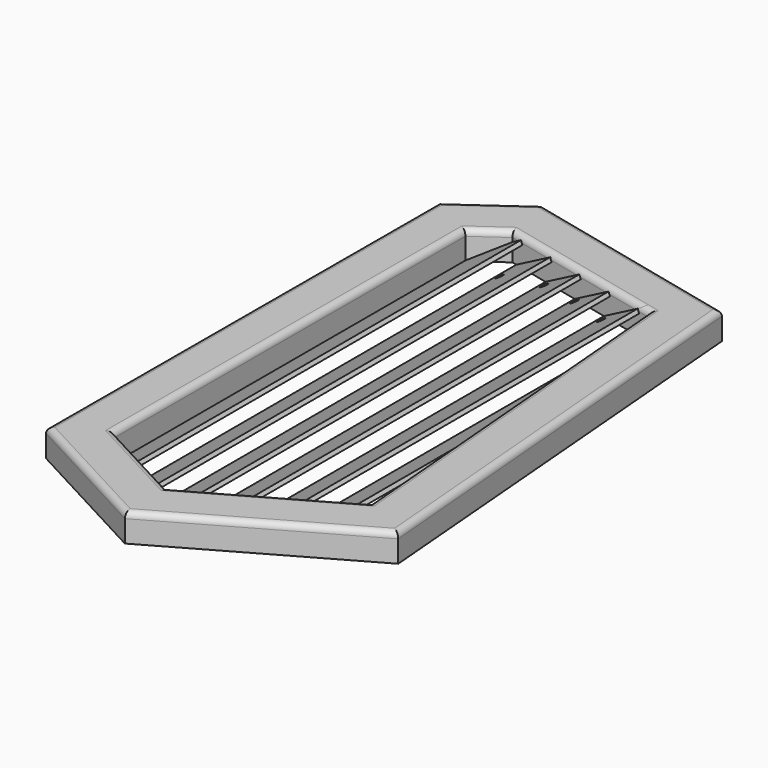
from build123d import *

# Parameters (mm, degrees)
F1_W           = 1
F1_H           = 127.4104844779
F2_DEPTH       = 12
F1_H_2         = 132.846667897
F1_H_3         = 133.8659538887
F1_H_4         = 125.3719197121
F1_H_5         = 118.236936396
F1_H_6         = 128.7695337087
F3_ANGLE       = -60
F4_ANGLE       = -60
F5_ANGLE       = -60
F6_ANGLE       = -60
F7_ANGLE       = -60
F8_ANGLE       = -60
F10_D          = 2
F12_D          = 2
F14_D          = 2
F16_D          = 2
F18_D          = 2
F19_DEPTH      = 7
F20_T1_DEPTH   = 64.3707659931
F20_T3_DEPTH   = 27.8907851503
F20_T5_DEPTH   = 130.1079313017
F20_T7_DEPTH   = 46.7691989997
F20_T9_DEPTH   = 61.7403046628
F20_T11_DEPTH  = 121.2232351314
F20_T16_DEPTH  = 47.9519770563
F20_T22_DEPTH  = 47.9519770563
F20_T28_DEPTH  = 47.9519770563
F20_T34_DEPTH  = 47.9519770563
F20_T40_DEPTH  = 47.9519770563
F20_T46_DEPTH  = 33.4399000359
F20_T52_DEPTH  = 33.4399000359
F20_T58_DEPTH  = 33.4399000359
F20_T64_DEPTH  = 117.2163729424
F20_T70_DEPTH  = 16.7204599427
F20_T76_DEPTH  = 50.7233823642
F20_T82_DEPTH  = 50.7233823642
F20_T88_DEPTH  = 50.7233823642
F20_T94_DEPTH  = 50.7233823642
F20_T100_DEPTH = 50.7233823642
F20_T106_DEPTH = 50.7233823642
F20_T112_DEPTH = 105.3966809672
F20_T118_DEPTH = 105.3966809672
F20_T125_DEPTH = 47.9519770563
F20_T129_DEPTH = 105.3966809672
F20_T136_DEPTH = 33.4399000359
F20_T140_DEPTH = 47.9519770563
F20_T147_DEPTH = 117.2163729424
F20_T151_DEPTH = 33.4399000359
F20_T158_DEPTH = 117.2163729424
F20_T162_DEPTH = 16.7204599427
F20_T169_DEPTH = 50.7233823642
F20_T173_DEPTH = 16.7204599427
F20_T180_DEPTH = 50.7233823642
F20_T184_DEPTH = 105.3966809672


# Not quite as in the source:
# - a fillet or chamfer that OpenCascade refuses, or shapes differently, is made with other operations: its cross-section is extruded or revolved along the edge and cut away or added


with BuildPart() as f2:
    # F1 (on Top) → F2 (new body)
    with BuildSketch(Plane.XY):
        with Locations((0.5, -55.8595443144)):
            Rectangle(F1_W, F1_H)
    extrude(amount=F2_DEPTH)


with BuildPart() as f2b:
    # F1 (on Top) → F2, piece 2 (new body)
    with BuildSketch(Plane.XY):
        with Locations((9.5, -58.9173960034)):
            Rectangle(F1_W, F1_H_2)
    extrude(amount=F2_DEPTH)


with BuildPart() as f2c:
    # F1 (on Top) → F2, piece 3 (new body)
    with BuildSketch(Plane.XY):
        with Locations((18.5, -60.1065598894)):
            Rectangle(F1_W, F1_H_3)
    extrude(amount=F2_DEPTH)


with BuildPart() as f2d:
    # F1 (on Top) → F2, piece 4 (new body)
    with BuildSketch(Plane.XY):
        with Locations((36.5, -59.257156332)):
            Rectangle(F1_W, F1_H_4)
    extrude(amount=F2_DEPTH)


with BuildPart() as f2e:
    # F1 (on Top) → F2, piece 5 (new body)
    with BuildSketch(Plane.XY):
        with Locations((45.5, -56.7089506658)):
            Rectangle(F1_W, F1_H_5)
    extrude(amount=F2_DEPTH)


with BuildPart() as f2f:
    # F1 (on Top) → F2, piece 6 (new body)
    with BuildSketch(Plane.XY):
        with Locations((27.5, -59.2571562156)):
            Rectangle(F1_W, F1_H_6)
    extrude(amount=F2_DEPTH)


with BuildPart() as f2_1:
    # F3: moved
    add(f2.part.rotate(Axis((0, -55.8595443144, 0), (0, -1, 0)), F3_ANGLE))



with BuildPart() as f2b_1:
    # F4: moved
    add(f2b.part.rotate(Axis((9, -58.9173960034, 0), (0, -1, 0)), F4_ANGLE))

    # F10 (through all)
    with Locations(Plane(origin=(2.25, 0, -3.897114317), x_dir=(0.8660254038, 0, 0.5), z_dir=(-0.5, 0, 0.8660254038))):
        with Locations((9.7942286341, -112.9602642174), (9.7942286341, -2.9387139806)):
            Hole(F10_D / 2)


with BuildPart() as f2c_1:
    # F5: moved
    add(f2c.part.rotate(Axis((18, -60.1065598894, 0), (0, -1, 0)), F5_ANGLE))

    # F12 (through all)
    with Locations(Plane(origin=(4.5, 0, -7.7942286341), x_dir=(0.8660254038, 0, 0.5), z_dir=(-0.5, 0, 0.8660254038))):
        with Locations((18.324283883, -117.2249242663), (18.324283883, -0.9955040878)):
            Hole(F12_D / 2)


with BuildPart() as f2f_1:
    # F6: moved
    add(f2f.part.rotate(Axis((27, -59.2571562156, 0), (0, -1, 0)), F6_ANGLE))

    # F14 (through all)
    with Locations(Plane(origin=(6.75, 0, -11.6913429511), x_dir=(0.8660254038, 0, 0.5), z_dir=(-0.5, 0, 0.8660254038))):
        with Locations((25.7820524275, -2.3019914515), (26.0747242719, -116.0897985101)):
            Hole(F14_D / 2)


with BuildPart() as f2d_1:
    # F7: moved
    add(f2d.part.rotate(Axis((36, -59.257156332, 0), (0, -1, 0)), F7_ANGLE))

    # F16 (through all)
    with Locations(Plane(origin=(9, 0, -15.5884572681), x_dir=(0.8660254038, 0, 0.5), z_dir=(-0.5, 0, 0.8660254038))):
        with Locations((33.6682610214, -110.1817563176), (33.4965772927, -5.2406745963)):
            Hole(F16_D / 2)


with BuildPart() as f2e_1:
    # F8: moved
    add(f2e.part.rotate(Axis((45, -56.7089506658, 0), (0, -1, 0)), F8_ANGLE))

    # F18 (through all)
    with Locations(Plane(origin=(11.25, 0, -19.4855715851), x_dir=(0.8660254038, 0, 0.5), z_dir=(-0.5, 0, 0.8660254038))):
        with Locations((41.2861332297, -6.0908603482), (41.4609648287, -105.8669760823)):
            Hole(F18_D / 2)


with BuildPart() as f2_2:
    add(f2_1.part)

    add(f2b_1.part)  # F19 merges F2b

    add(f2c_1.part)  # F19 merges F2c

    add(f2d_1.part)  # F19 merges F2d

    add(f2e_1.part)  # F19 merges F2e

    add(f2f_1.part)  # F19 merges F2f
    # F0 (on Top) → F19 (join)
    with BuildSketch(Plane.XY):
        Polygon((5.3426049832, 17.2253030222), (-11.2654683454, 5.3950021233), (-11.5938979585, -117.2124892957), (23.0112235707, -135.7746969778), (70.1950419827, -109.0221656961), (60.7265483736, 4.3062148514), align=None)
        Polygon((22.856560841, -122.5590744219), (-0.0023194154, -110.2973450456), (0.2913901898, -0.5813652328), (7.8014298177, 4.7680446734), (49.894827921, -5.0506425668), (58.0459460053, -102.6073922993), align=None, mode=Mode.SUBTRACT)
    extrude(amount=F19_DEPTH)

    # F20: fillet of radius 1.5 on 12 edges, made by hand

    # F20_s2 → F20_t1 (cut)
    with BuildSketch(Plane(origin=(60.292110333, -14.0639875334, 0), x_dir=(0, 0, 1), z_dir=(-0.9738561179, 0.2271657141, 0))):
        with BuildLine():
            ThreePointArc((5.5, 17.9886234068), (6.5606601718, 17.5492835785), (7, 16.4886234068))
            Line((7, 16.4886234068), (7, 17.9886234068))
            Line((7, 17.9886234068), (5.5, 17.9886234068))
        make_face()
    extrude(amount=F20_T1_DEPTH, mode=Mode.SUBTRACT)

    # F20_s4 → F20_t3 (cut)
    with BuildSketch(Plane(origin=(14.7383841481, 10.498479612, 0), x_dir=(0, 0, 1), z_dir=(-0.8144891531, -0.5801787823, 0))):
        with BuildLine():
            ThreePointArc((5.5, 10.9301564173), (6.5606601718, 10.4908165891), (7, 9.4301564173))
            Line((7, 9.4301564173), (7, 10.9301564173))
            Line((7, 10.9301564173), (5.5, 10.9301564173))
        make_face()
    extrude(amount=F20_T3_DEPTH, mode=Mode.SUBTRACT)

    # F20_s6 → F20_t5 (cut)
    with BuildSketch(Plane(origin=(0.024415812, 9.1147732794, 0), x_dir=(0, 0, 1), z_dir=(-0.0026786979, -0.9999964123, 0))):
        with BuildLine():
            ThreePointArc((5.5, 11.2798795092), (6.5606601718, 10.840539681), (7, 9.7798795092))
            Line((7, 9.7798795092), (7, 11.2798795092))
            Line((7, 11.2798795092), (5.5, 11.2798795092))
        make_face()
    extrude(amount=F20_T5_DEPTH, mode=Mode.SUBTRACT)

    # F20_s8 → F20_t7 (cut)
    with BuildSketch(Plane(origin=(36.516728388, -19.5875947333, 0), x_dir=(0, 0, 1), z_dir=(0.8812280976, -0.4726912734, 0))):
        with BuildLine():
            ThreePointArc((5.5, 108.7712733481), (6.5606601718, 108.3319335199), (7, 107.2712733481))
            Line((7, 107.2712733481), (7, 108.7712733481))
            Line((7, 108.7712733481), (5.5, 108.7712733481))
        make_face()
    extrude(amount=F20_T7_DEPTH, mode=Mode.SUBTRACT)

    # F20_s10 → F20_t9 (cut)
    with BuildSketch(Plane(origin=(-44.1037290174, -25.0061658825, 0), x_dir=(0, 0, 1), z_dir=(0.8699032704, 0.4932223639, 0))):
        with BuildLine():
            ThreePointArc((5.5, 129.4605030189), (6.5606601718, 129.0211631907), (7, 127.9605030189))
            Line((7, 127.9605030189), (7, 129.4605030189))
            Line((7, 129.4605030189), (5.5, 129.4605030189))
        make_face()
    extrude(amount=F20_T9_DEPTH, mode=Mode.SUBTRACT)

    # F20_s12 → F20_t11 (cut)
    with BuildSketch(Plane(origin=(9.8443896099, -117.8274790096, 0), x_dir=(0, 0, 1), z_dir=(-0.0832590947, 0.9965279339, 0))):
        with BuildLine():
            ThreePointArc((5.5, 60.874233337), (6.5606601718, 60.4348935088), (7, 59.374233337))
            Line((7, 59.374233337), (7, 60.874233337))
            Line((7, 60.874233337), (5.5, 60.874233337))
        make_face()
    extrude(amount=F20_T11_DEPTH, mode=Mode.SUBTRACT)


with BuildPart() as f20_tool14:
    # F20_s15 → F20_t16 (new body)
    with BuildSketch(Plane(origin=(3.1634613529, 1.7936197244, 0), x_dir=(0, 0, 1), z_dir=(-0.8699051993, -0.4932189617, 0))):
        with BuildLine():
            ThreePointArc((5.5, -117.8880652704), (6.5606601718, -118.3274050986), (7, -119.3880652704))
            Line((7, -119.3880652704), (7, -117.8880652704))
            Line((7, -117.8880652704), (5.5, -117.8880652704))
        make_face()
    extrude(amount=F20_T16_DEPTH)

    split(bisect_by=Plane(origin=(49.1298565306, 4.1049262418, 0), x_dir=(0, 0, 1), z_dir=(-0.9965276531, -0.0832624559, 0)), keep=Keep.TOP)

    split(bisect_by=Plane(origin=(44.1423048454, 0, 25.4855715851), x_dir=(0, 1, 0), z_dir=(0.8660254038, 0, 0.5)), keep=Keep.TOP)


with BuildPart() as f2_3:
    add(f2_2.part)

    # F20_t13: cut F20_tool14
    add(f20_tool14.part, mode=Mode.SUBTRACT)


with BuildPart() as f20_tool20:
    # F20_s21 → F20_t22 (new body)
    with BuildSketch(Plane(origin=(3.1634613529, 1.7936197244, 0), x_dir=(0, 0, 1), z_dir=(-0.8699051993, -0.4932189617, 0))):
        with BuildLine():
            ThreePointArc((5.5, -117.8880652704), (6.5606601718, -118.3274050986), (7, -119.3880652704))
            Line((7, -119.3880652704), (7, -117.8880652704))
            Line((7, -117.8880652704), (5.5, -117.8880652704))
        make_face()
    extrude(amount=F20_T22_DEPTH)

    split(bisect_by=Plane(origin=(37.3923048454, 0, 21.5884572681), x_dir=(0, 1, 0), z_dir=(0.8660254038, 0, 0.5)), keep=Keep.TOP)

    split(bisect_by=Plane(origin=(11.25, 0, -19.4855715851), x_dir=(0, 1, 0), z_dir=(-0.5, 0, 0.8660254038)), keep=Keep.TOP)


with BuildPart() as f2_4:
    add(f2_3.part)

    # F20_t19: cut F20_tool20
    add(f20_tool20.part, mode=Mode.SUBTRACT)


with BuildPart() as f20_tool26:
    # F20_s27 → F20_t28 (new body)
    with BuildSketch(Plane(origin=(3.1634613529, 1.7936197244, 0), x_dir=(0, 0, 1), z_dir=(-0.8699051993, -0.4932189617, 0))):
        with BuildLine():
            ThreePointArc((5.5, -117.8880652704), (6.5606601718, -118.3274050986), (7, -119.3880652704))
            Line((7, -119.3880652704), (7, -117.8880652704))
            Line((7, -117.8880652704), (5.5, -117.8880652704))
        make_face()
    extrude(amount=F20_T28_DEPTH)

    split(bisect_by=Plane(origin=(30.6423048454, 0, 17.6913429511), x_dir=(0, 1, 0), z_dir=(0.8660254038, 0, 0.5)), keep=Keep.TOP)

    split(bisect_by=Plane(origin=(9, 0, -15.5884572681), x_dir=(0, 1, 0), z_dir=(-0.5, 0, 0.8660254038)), keep=Keep.TOP)


with BuildPart() as f2_5:
    add(f2_4.part)

    # F20_t25: cut F20_tool26
    add(f20_tool26.part, mode=Mode.SUBTRACT)


with BuildPart() as f20_tool32:
    # F20_s33 → F20_t34 (new body)
    with BuildSketch(Plane(origin=(3.1634613529, 1.7936197244, 0), x_dir=(0, 0, 1), z_dir=(-0.8699051993, -0.4932189617, 0))):
        with BuildLine():
            ThreePointArc((5.5, -117.8880652704), (6.5606601718, -118.3274050986), (7, -119.3880652704))
            Line((7, -119.3880652704), (7, -117.8880652704))
            Line((7, -117.8880652704), (5.5, -117.8880652704))
        make_face()
    extrude(amount=F20_T34_DEPTH)

    split(bisect_by=Plane(origin=(6.75, 0, -11.6913429511), x_dir=(0, 1, 0), z_dir=(-0.5, 0, 0.8660254038)), keep=Keep.TOP)

    split(bisect_by=Plane(origin=(23.8923048454, 0, 13.7942286341), x_dir=(0, 1, 0), z_dir=(0.8660254038, 0, 0.5)), keep=Keep.TOP)


with BuildPart() as f2_6:
    add(f2_5.part)

    # F20_t31: cut F20_tool32
    add(f20_tool32.part, mode=Mode.SUBTRACT)


with BuildPart() as f20_tool38:
    # F20_s39 → F20_t40 (new body)
    with BuildSketch(Plane(origin=(3.1634613529, 1.7936197244, 0), x_dir=(0, 0, 1), z_dir=(-0.8699051993, -0.4932189617, 0))):
        with BuildLine():
            ThreePointArc((5.5, -117.8880652704), (6.5606601718, -118.3274050986), (7, -119.3880652704))
            Line((7, -119.3880652704), (7, -117.8880652704))
            Line((7, -117.8880652704), (5.5, -117.8880652704))
        make_face()
    extrude(amount=F20_T40_DEPTH)

    split(bisect_by=Plane(origin=(-45.9451888224, -85.6531356567, 0), x_dir=(0, 0, 1), z_dir=(0.4726976341, 0.8812246857, 0)), keep=Keep.TOP)

    split(bisect_by=Plane(origin=(4.5, 0, -7.7942286341), x_dir=(0, 1, 0), z_dir=(-0.5, 0, 0.8660254038)), keep=Keep.TOP)


with BuildPart() as f2_7:
    add(f2_6.part)

    # F20_t37: cut F20_tool38
    add(f20_tool38.part, mode=Mode.SUBTRACT)


with BuildPart() as f20_tool44:
    # F20_s45 → F20_t46 (new body)
    with BuildSketch(Plane(origin=(72.1063422347, -38.6785548931, 0), x_dir=(0, 0, 1), z_dir=(-0.8812246857, 0.4726976341, 0))):
        with BuildLine():
            ThreePointArc((5.5, -97.1978396043), (6.5606601718, -97.6371794325), (7, -98.6978396043))
            Line((7, -98.6978396043), (7, -97.1978396043))
            Line((7, -97.1978396043), (5.5, -97.1978396043))
        make_face()
    extrude(amount=F20_T46_DEPTH)

    split(bisect_by=Plane(origin=(58.1446291498, -102.5514409174, 0), x_dir=(0, 0, 1), z_dir=(-0.4932189617, 0.8699051993, 0)), keep=Keep.TOP)

    split(bisect_by=Plane(origin=(17.1423048454, 0, 9.897114317), x_dir=(0, 1, 0), z_dir=(0.8660254038, 0, 0.5)), keep=Keep.TOP)


with BuildPart() as f2_8:
    add(f2_7.part)

    # F20_t43: cut F20_tool44
    add(f20_tool44.part, mode=Mode.SUBTRACT)


with BuildPart() as f20_tool50:
    # F20_s51 → F20_t52 (new body)
    with BuildSketch(Plane(origin=(72.1063422347, -38.6785548931, 0), x_dir=(0, 0, 1), z_dir=(-0.8812246857, 0.4726976341, 0))):
        with BuildLine():
            ThreePointArc((5.5, -97.1978396043), (6.5606601718, -97.6371794325), (7, -98.6978396043))
            Line((7, -98.6978396043), (7, -97.1978396043))
            Line((7, -97.1978396043), (5.5, -97.1978396043))
        make_face()
    extrude(amount=F20_T52_DEPTH)

    split(bisect_by=Plane(origin=(2.25, 0, -3.897114317), x_dir=(0, 1, 0), z_dir=(-0.5, 0, 0.8660254038)), keep=Keep.TOP)

    split(bisect_by=Plane(origin=(10.3923048454, 0, 6), x_dir=(0, 1, 0), z_dir=(0.8660254038, 0, 0.5)), keep=Keep.TOP)


with BuildPart() as f2_9:
    add(f2_8.part)

    # F20_t49: cut F20_tool50
    add(f20_tool50.part, mode=Mode.SUBTRACT)


with BuildPart() as f20_tool56:
    # F20_s57 → F20_t58 (new body)
    with BuildSketch(Plane(origin=(72.1063422347, -38.6785548931, 0), x_dir=(0, 0, 1), z_dir=(-0.8812246857, 0.4726976341, 0))):
        with BuildLine():
            ThreePointArc((5.5, -97.1978396043), (6.5606601718, -97.6371794325), (7, -98.6978396043))
            Line((7, -98.6978396043), (7, -97.1978396043))
            Line((7, -97.1978396043), (5.5, -97.1978396043))
        make_face()
    extrude(amount=F20_T58_DEPTH)

    split(bisect_by=Plane(origin=(0.2929444048, -0.000784212, 0), x_dir=(0, 0, 1), z_dir=(0.9999964169, -0.0026769897, 0)), keep=Keep.TOP)

    split(bisect_by=Plane(origin=(0, 0, 0), x_dir=(0, 1, 0), z_dir=(-0.5, 0, 0.8660254038)), keep=Keep.TOP)


with BuildPart() as f2_10:
    add(f2_9.part)

    # F20_t55: cut F20_tool56
    add(f20_tool56.part, mode=Mode.SUBTRACT)


with BuildPart() as f20_tool62:
    # F20_s63 → F20_t64 (new body)
    with BuildSketch(Plane(origin=(-0.3053025318, -114.0465473969, 0), x_dir=(0, 0, 1), z_dir=(0.0026769897, 0.9999964169, 0))):
        with BuildLine():
            ThreePointArc((5.5, 0.2929454545), (6.5606601718, -0.1463943737), (7, -1.2070545455))
            Line((7, -1.2070545455), (7, 0.2929454545))
            Line((7, 0.2929454545), (5.5, 0.2929454545))
        make_face()
    extrude(amount=F20_T64_DEPTH)

    split(bisect_by=Plane(origin=(-45.9451888224, -85.6531356567, 0), x_dir=(0, 0, 1), z_dir=(0.4726976341, 0.8812246857, 0)), keep=Keep.TOP)

    split(bisect_by=Plane(origin=(0.372801322, -0.5233759892, 0), x_dir=(0, 0, 1), z_dir=(0.5801673603, -0.8144972891, 0)), keep=Keep.TOP)


with BuildPart() as f2_11:
    add(f2_10.part)

    # F20_t61: cut F20_tool62
    add(f20_tool62.part, mode=Mode.SUBTRACT)


with BuildPart() as f20_tool68:
    # F20_s69 → F20_t70 (new body)
    with BuildSketch(Plane(origin=(-3.1357759664, -2.2336168448, 0), x_dir=(0, 0, 1), z_dir=(0.8144972891, 0.5801673603, 0))):
        with BuildLine():
            ThreePointArc((7, -0.8574245167), (6.5606601718, 0.2032356551), (5.5, 0.6425754833))
            Line((5.5, 0.6425754833), (7, 0.6425754833))
            Line((7, 0.6425754833), (7, -0.8574245167))
        make_face()
    extrude(amount=F20_T70_DEPTH)

    split(bisect_by=Plane(origin=(1.4573722643, 6.2478567046, 0), x_dir=(0, 0, 1), z_dir=(-0.2271614738, -0.973857107, 0)), keep=Keep.TOP)

    split(bisect_by=Plane(origin=(0.2929444048, -0.000784212, 0), x_dir=(0, 0, 1), z_dir=(0.9999964169, -0.0026769897, 0)), keep=Keep.TOP)


with BuildPart() as f2_12:
    add(f2_11.part)

    # F20_t67: cut F20_tool68
    add(f20_tool68.part, mode=Mode.SUBTRACT)


with BuildPart() as f20_tool74:
    # F20_s75 → F20_t76 (new body)
    with BuildSketch(Plane(origin=(2.6920934022, -0.6279565046, 0), x_dir=(0, 0, 1), z_dir=(0.973857107, -0.2271614738, 0))):
        with BuildLine():
            ThreePointArc((5.5, -6.4155784866), (6.5606601718, -6.8549183149), (7, -7.9155784866))
            Line((7, -7.9155784866), (7, -6.4155784866))
            Line((7, -6.4155784866), (5.5, -6.4155784866))
        make_face()
    extrude(amount=F20_T76_DEPTH)

    split(bisect_by=Plane(origin=(0.372801322, -0.5233759892, 0), x_dir=(0, 0, 1), z_dir=(0.5801673603, -0.8144972891, 0)), keep=Keep.TOP)

    split(bisect_by=Plane(origin=(0, 0, 0), x_dir=(0, 1, 0), z_dir=(-0.5, 0, 0.8660254038)), keep=Keep.TOP)


with BuildPart() as f2_13:
    add(f2_12.part)

    # F20_t73: cut F20_tool74
    add(f20_tool74.part, mode=Mode.SUBTRACT)


with BuildPart() as f20_tool80:
    # F20_s81 → F20_t82 (new body)
    with BuildSketch(Plane(origin=(2.6920934022, -0.6279565046, 0), x_dir=(0, 0, 1), z_dir=(0.973857107, -0.2271614738, 0))):
        with BuildLine():
            ThreePointArc((5.5, -6.4155784866), (6.5606601718, -6.8549183149), (7, -7.9155784866))
            Line((7, -7.9155784866), (7, -6.4155784866))
            Line((7, -6.4155784866), (5.5, -6.4155784866))
        make_face()
    extrude(amount=F20_T82_DEPTH)

    split(bisect_by=Plane(origin=(2.25, 0, -3.897114317), x_dir=(0, 1, 0), z_dir=(-0.5, 0, 0.8660254038)), keep=Keep.TOP)

    split(bisect_by=Plane(origin=(10.3923048454, 0, 6), x_dir=(0, 1, 0), z_dir=(0.8660254038, 0, 0.5)), keep=Keep.TOP)


with BuildPart() as f2_14:
    add(f2_13.part)

    # F20_t79: cut F20_tool80
    add(f20_tool80.part, mode=Mode.SUBTRACT)


with BuildPart() as f20_tool86:
    # F20_s87 → F20_t88 (new body)
    with BuildSketch(Plane(origin=(2.6920934022, -0.6279565046, 0), x_dir=(0, 0, 1), z_dir=(0.973857107, -0.2271614738, 0))):
        with BuildLine():
            ThreePointArc((5.5, -6.4155784866), (6.5606601718, -6.8549183149), (7, -7.9155784866))
            Line((7, -7.9155784866), (7, -6.4155784866))
            Line((7, -6.4155784866), (5.5, -6.4155784866))
        make_face()
    extrude(amount=F20_T88_DEPTH)

    split(bisect_by=Plane(origin=(17.1423048454, 0, 9.897114317), x_dir=(0, 1, 0), z_dir=(0.8660254038, 0, 0.5)), keep=Keep.TOP)

    split(bisect_by=Plane(origin=(4.5, 0, -7.7942286341), x_dir=(0, 1, 0), z_dir=(-0.5, 0, 0.8660254038)), keep=Keep.TOP)


with BuildPart() as f2_15:
    add(f2_14.part)

    # F20_t85: cut F20_tool86
    add(f20_tool86.part, mode=Mode.SUBTRACT)


with BuildPart() as f20_tool92:
    # F20_s93 → F20_t94 (new body)
    with BuildSketch(Plane(origin=(2.6920934022, -0.6279565046, 0), x_dir=(0, 0, 1), z_dir=(0.973857107, -0.2271614738, 0))):
        with BuildLine():
            ThreePointArc((5.5, -6.4155784866), (6.5606601718, -6.8549183149), (7, -7.9155784866))
            Line((7, -7.9155784866), (7, -6.4155784866))
            Line((7, -6.4155784866), (5.5, -6.4155784866))
        make_face()
    extrude(amount=F20_T94_DEPTH)

    split(bisect_by=Plane(origin=(6.75, 0, -11.6913429511), x_dir=(0, 1, 0), z_dir=(-0.5, 0, 0.8660254038)), keep=Keep.TOP)

    split(bisect_by=Plane(origin=(23.8923048454, 0, 13.7942286341), x_dir=(0, 1, 0), z_dir=(0.8660254038, 0, 0.5)), keep=Keep.TOP)


with BuildPart() as f2_16:
    add(f2_15.part)

    # F20_t91: cut F20_tool92
    add(f20_tool92.part, mode=Mode.SUBTRACT)


with BuildPart() as f20_tool98:
    # F20_s99 → F20_t100 (new body)
    with BuildSketch(Plane(origin=(2.6920934022, -0.6279565046, 0), x_dir=(0, 0, 1), z_dir=(0.973857107, -0.2271614738, 0))):
        with BuildLine():
            ThreePointArc((5.5, -6.4155784866), (6.5606601718, -6.8549183149), (7, -7.9155784866))
            Line((7, -7.9155784866), (7, -6.4155784866))
            Line((7, -6.4155784866), (5.5, -6.4155784866))
        make_face()
    extrude(amount=F20_T100_DEPTH)

    split(bisect_by=Plane(origin=(30.6423048454, 0, 17.6913429511), x_dir=(0, 1, 0), z_dir=(0.8660254038, 0, 0.5)), keep=Keep.TOP)

    split(bisect_by=Plane(origin=(9, 0, -15.5884572681), x_dir=(0, 1, 0), z_dir=(-0.5, 0, 0.8660254038)), keep=Keep.TOP)


with BuildPart() as f2_17:
    add(f2_16.part)

    # F20_t97: cut F20_tool98
    add(f20_tool98.part, mode=Mode.SUBTRACT)


with BuildPart() as f20_tool104:
    # F20_s105 → F20_t106 (new body)
    with BuildSketch(Plane(origin=(2.6920934022, -0.6279565046, 0), x_dir=(0, 0, 1), z_dir=(0.973857107, -0.2271614738, 0))):
        with BuildLine():
            ThreePointArc((5.5, -6.4155784866), (6.5606601718, -6.8549183149), (7, -7.9155784866))
            Line((7, -7.9155784866), (7, -6.4155784866))
            Line((7, -6.4155784866), (5.5, -6.4155784866))
        make_face()
    extrude(amount=F20_T106_DEPTH)

    split(bisect_by=Plane(origin=(49.1298565306, 4.1049262418, 0), x_dir=(0, 0, 1), z_dir=(-0.9965276531, -0.0832624559, 0)), keep=Keep.TOP)

    split(bisect_by=Plane(origin=(37.3923048454, 0, 21.5884572681), x_dir=(0, 1, 0), z_dir=(0.8660254038, 0, 0.5)), keep=Keep.TOP)


with BuildPart() as f2_18:
    add(f2_17.part)

    # F20_t103: cut F20_tool104
    add(f20_tool104.part, mode=Mode.SUBTRACT)


with BuildPart() as f20_tool110:
    # F20_s111 → F20_t112 (new body)
    with BuildSketch(Plane(origin=(0.4527371807, -5.4185901095, 0), x_dir=(0, 0, 1), z_dir=(0.0832624559, -0.9965276531, 0))):
        with BuildLine():
            ThreePointArc((5.5, -49.3010468668), (6.5606601718, -49.740386695), (7, -50.8010468668))
            Line((7, -50.8010468668), (7, -49.3010468668))
            Line((7, -49.3010468668), (5.5, -49.3010468668))
        make_face()
    extrude(amount=F20_T112_DEPTH)

    split(bisect_by=Plane(origin=(1.4573722643, 6.2478567046, 0), x_dir=(0, 0, 1), z_dir=(-0.2271614738, -0.973857107, 0)), keep=Keep.TOP)

    split(bisect_by=Plane(origin=(11.25, 0, -19.4855715851), x_dir=(0, 1, 0), z_dir=(-0.5, 0, 0.8660254038)), keep=Keep.TOP)


with BuildPart() as f2_19:
    add(f2_18.part)

    # F20_t109: cut F20_tool110
    add(f20_tool110.part, mode=Mode.SUBTRACT)


with BuildPart() as f20_tool116:
    # F20_s117 → F20_t118 (new body)
    with BuildSketch(Plane(origin=(0.4527371807, -5.4185901095, 0), x_dir=(0, 0, 1), z_dir=(0.0832624559, -0.9965276531, 0))):
        with BuildLine():
            ThreePointArc((5.5, -49.3010468668), (6.5606601718, -49.740386695), (7, -50.8010468668))
            Line((7, -50.8010468668), (7, -49.3010468668))
            Line((7, -49.3010468668), (5.5, -49.3010468668))
        make_face()
    extrude(amount=F20_T118_DEPTH)

    split(bisect_by=Plane(origin=(58.1446291498, -102.5514409174, 0), x_dir=(0, 0, 1), z_dir=(-0.4932189617, 0.8699051993, 0)), keep=Keep.TOP)

    split(bisect_by=Plane(origin=(44.1423048454, 0, 25.4855715851), x_dir=(0, 1, 0), z_dir=(0.8660254038, 0, 0.5)), keep=Keep.TOP)


with BuildPart() as f2_20:
    add(f2_19.part)

    # F20_t115: cut F20_tool116
    add(f20_tool116.part, mode=Mode.SUBTRACT)


with BuildPart() as f20_tool123:
    # F20_s124 → F20_t125 (new body)
    with BuildSketch(Plane(origin=(3.1634613529, 1.7936197244, 0), x_dir=(0, 0, 1), z_dir=(-0.8699051993, -0.4932189617, 0))):
        with BuildLine():
            ThreePointArc((5.5, -117.8880652704), (6.5606601718, -118.3274050986), (7, -119.3880652704))
            Line((7, -119.3880652704), (7, -117.8880652704))
            Line((7, -117.8880652704), (5.5, -117.8880652704))
        make_face()
    extrude(amount=F20_T125_DEPTH)

    split(bisect_by=Plane(origin=(49.1298565306, 4.1049262418, 0), x_dir=(0, 0, 1), z_dir=(0.9965276531, 0.0832624559, 0)), keep=Keep.TOP)


with BuildPart() as f20_tool127:
    # F20_s128 → F20_t129 (new body)
    with BuildSketch(Plane(origin=(0.4527371807, -5.4185901095, 0), x_dir=(0, 0, 1), z_dir=(0.0832624559, -0.9965276531, 0))):
        with BuildLine():
            ThreePointArc((5.5, -49.3010468668), (6.5606601718, -49.740386695), (7, -50.8010468668))
            Line((7, -50.8010468668), (7, -49.3010468668))
            Line((7, -49.3010468668), (5.5, -49.3010468668))
        make_face()
    extrude(amount=F20_T129_DEPTH)

    split(bisect_by=Plane(origin=(58.1446291498, -102.5514409174, 0), x_dir=(0, 0, 1), z_dir=(0.4932189617, -0.8699051993, 0)), keep=Keep.TOP)


with BuildPart() as f20_tool123_1:
    add(f20_tool123.part)

    # F20_t131: intersect F20_tool127
    add(f20_tool127.part, mode=Mode.INTERSECT)


with BuildPart() as f2_21:
    add(f2_20.part)

    # F20_t121: cut F20_tool123
    add(f20_tool123_1.part, mode=Mode.SUBTRACT)


with BuildPart() as f20_tool134:
    # F20_s135 → F20_t136 (new body)
    with BuildSketch(Plane(origin=(72.1063422347, -38.6785548931, 0), x_dir=(0, 0, 1), z_dir=(-0.8812246857, 0.4726976341, 0))):
        with BuildLine():
            ThreePointArc((5.5, -97.1978396043), (6.5606601718, -97.6371794325), (7, -98.6978396043))
            Line((7, -98.6978396043), (7, -97.1978396043))
            Line((7, -97.1978396043), (5.5, -97.1978396043))
        make_face()
    extrude(amount=F20_T136_DEPTH)

    split(bisect_by=Plane(origin=(58.1446291498, -102.5514409174, 0), x_dir=(0, 0, 1), z_dir=(0.4932189617, -0.8699051993, 0)), keep=Keep.TOP)


with BuildPart() as f20_tool138:
    # F20_s139 → F20_t140 (new body)
    with BuildSketch(Plane(origin=(3.1634613529, 1.7936197244, 0), x_dir=(0, 0, 1), z_dir=(-0.8699051993, -0.4932189617, 0))):
        with BuildLine():
            ThreePointArc((5.5, -117.8880652704), (6.5606601718, -118.3274050986), (7, -119.3880652704))
            Line((7, -119.3880652704), (7, -117.8880652704))
            Line((7, -117.8880652704), (5.5, -117.8880652704))
        make_face()
    extrude(amount=F20_T140_DEPTH)

    split(bisect_by=Plane(origin=(-45.9451888224, -85.6531356567, 0), x_dir=(0, 0, 1), z_dir=(-0.4726976341, -0.8812246857, 0)), keep=Keep.TOP)


with BuildPart() as f20_tool134_1:
    add(f20_tool134.part)

    # F20_t142: intersect F20_tool138
    add(f20_tool138.part, mode=Mode.INTERSECT)


with BuildPart() as f2_22:
    add(f2_21.part)

    # F20_t132: cut F20_tool134
    add(f20_tool134_1.part, mode=Mode.SUBTRACT)


with BuildPart() as f20_tool145:
    # F20_s146 → F20_t147 (new body)
    with BuildSketch(Plane(origin=(-0.3053025318, -114.0465473969, 0), x_dir=(0, 0, 1), z_dir=(0.0026769897, 0.9999964169, 0))):
        with BuildLine():
            ThreePointArc((5.5, 0.2929454545), (6.5606601718, -0.1463943737), (7, -1.2070545455))
            Line((7, -1.2070545455), (7, 0.2929454545))
            Line((7, 0.2929454545), (5.5, 0.2929454545))
        make_face()
    extrude(amount=F20_T147_DEPTH)

    split(bisect_by=Plane(origin=(-45.9451888224, -85.6531356567, 0), x_dir=(0, 0, 1), z_dir=(-0.4726976341, -0.8812246857, 0)), keep=Keep.TOP)


with BuildPart() as f20_tool149:
    # F20_s150 → F20_t151 (new body)
    with BuildSketch(Plane(origin=(72.1063422347, -38.6785548931, 0), x_dir=(0, 0, 1), z_dir=(-0.8812246857, 0.4726976341, 0))):
        with BuildLine():
            ThreePointArc((5.5, -97.1978396043), (6.5606601718, -97.6371794325), (7, -98.6978396043))
            Line((7, -98.6978396043), (7, -97.1978396043))
            Line((7, -97.1978396043), (5.5, -97.1978396043))
        make_face()
    extrude(amount=F20_T151_DEPTH)

    split(bisect_by=Plane(origin=(0.2929444048, -0.000784212, 0), x_dir=(0, 0, 1), z_dir=(-0.9999964169, 0.0026769897, 0)), keep=Keep.TOP)


with BuildPart() as f20_tool145_1:
    add(f20_tool145.part)

    # F20_t153: intersect F20_tool149
    add(f20_tool149.part, mode=Mode.INTERSECT)


with BuildPart() as f2_23:
    add(f2_22.part)

    # F20_t143: cut F20_tool145
    add(f20_tool145_1.part, mode=Mode.SUBTRACT)


with BuildPart() as f20_tool156:
    # F20_s157 → F20_t158 (new body)
    with BuildSketch(Plane(origin=(-0.3053025318, -114.0465473969, 0), x_dir=(0, 0, 1), z_dir=(0.0026769897, 0.9999964169, 0))):
        with BuildLine():
            ThreePointArc((5.5, 0.2929454545), (6.5606601718, -0.1463943737), (7, -1.2070545455))
            Line((7, -1.2070545455), (7, 0.2929454545))
            Line((7, 0.2929454545), (5.5, 0.2929454545))
        make_face()
    extrude(amount=F20_T158_DEPTH)

    split(bisect_by=Plane(origin=(0.372801322, -0.5233759892, 0), x_dir=(0, 0, 1), z_dir=(-0.5801673603, 0.8144972891, 0)), keep=Keep.TOP)


with BuildPart() as f20_tool160:
    # F20_s161 → F20_t162 (new body)
    with BuildSketch(Plane(origin=(-3.1357759664, -2.2336168448, 0), x_dir=(0, 0, 1), z_dir=(0.8144972891, 0.5801673603, 0))):
        with BuildLine():
            ThreePointArc((7, -0.8574245167), (6.5606601718, 0.2032356551), (5.5, 0.6425754833))
            Line((5.5, 0.6425754833), (7, 0.6425754833))
            Line((7, 0.6425754833), (7, -0.8574245167))
        make_face()
    extrude(amount=F20_T162_DEPTH)

    split(bisect_by=Plane(origin=(0.2929444048, -0.000784212, 0), x_dir=(0, 0, 1), z_dir=(-0.9999964169, 0.0026769897, 0)), keep=Keep.TOP)


with BuildPart() as f20_tool156_1:
    add(f20_tool156.part)

    # F20_t164: intersect F20_tool160
    add(f20_tool160.part, mode=Mode.INTERSECT)


with BuildPart() as f2_24:
    add(f2_23.part)

    # F20_t154: cut F20_tool156
    add(f20_tool156_1.part, mode=Mode.SUBTRACT)


with BuildPart() as f20_tool167:
    # F20_s168 → F20_t169 (new body)
    with BuildSketch(Plane(origin=(2.6920934022, -0.6279565046, 0), x_dir=(0, 0, 1), z_dir=(0.973857107, -0.2271614738, 0))):
        with BuildLine():
            ThreePointArc((5.5, -6.4155784866), (6.5606601718, -6.8549183149), (7, -7.9155784866))
            Line((7, -7.9155784866), (7, -6.4155784866))
            Line((7, -6.4155784866), (5.5, -6.4155784866))
        make_face()
    extrude(amount=F20_T169_DEPTH)

    split(bisect_by=Plane(origin=(0.372801322, -0.5233759892, 0), x_dir=(0, 0, 1), z_dir=(-0.5801673603, 0.8144972891, 0)), keep=Keep.TOP)


with BuildPart() as f20_tool171:
    # F20_s172 → F20_t173 (new body)
    with BuildSketch(Plane(origin=(-3.1357759664, -2.2336168448, 0), x_dir=(0, 0, 1), z_dir=(0.8144972891, 0.5801673603, 0))):
        with BuildLine():
            ThreePointArc((7, -0.8574245167), (6.5606601718, 0.2032356551), (5.5, 0.6425754833))
            Line((5.5, 0.6425754833), (7, 0.6425754833))
            Line((7, 0.6425754833), (7, -0.8574245167))
        make_face()
    extrude(amount=F20_T173_DEPTH)

    split(bisect_by=Plane(origin=(1.4573722643, 6.2478567046, 0), x_dir=(0, 0, 1), z_dir=(0.2271614738, 0.973857107, 0)), keep=Keep.TOP)


with BuildPart() as f20_tool167_1:
    add(f20_tool167.part)

    # F20_t175: intersect F20_tool171
    add(f20_tool171.part, mode=Mode.INTERSECT)


with BuildPart() as f2_25:
    add(f2_24.part)

    # F20_t165: cut F20_tool167
    add(f20_tool167_1.part, mode=Mode.SUBTRACT)


with BuildPart() as f20_tool178:
    # F20_s179 → F20_t180 (new body)
    with BuildSketch(Plane(origin=(2.6920934022, -0.6279565046, 0), x_dir=(0, 0, 1), z_dir=(0.973857107, -0.2271614738, 0))):
        with BuildLine():
            ThreePointArc((5.5, -6.4155784866), (6.5606601718, -6.8549183149), (7, -7.9155784866))
            Line((7, -7.9155784866), (7, -6.4155784866))
            Line((7, -6.4155784866), (5.5, -6.4155784866))
        make_face()
    extrude(amount=F20_T180_DEPTH)

    split(bisect_by=Plane(origin=(49.1298565306, 4.1049262418, 0), x_dir=(0, 0, 1), z_dir=(0.9965276531, 0.0832624559, 0)), keep=Keep.TOP)


with BuildPart() as f20_tool182:
    # F20_s183 → F20_t184 (new body)
    with BuildSketch(Plane(origin=(0.4527371807, -5.4185901095, 0), x_dir=(0, 0, 1), z_dir=(0.0832624559, -0.9965276531, 0))):
        with BuildLine():
            ThreePointArc((5.5, -49.3010468668), (6.5606601718, -49.740386695), (7, -50.8010468668))
            Line((7, -50.8010468668), (7, -49.3010468668))
            Line((7, -49.3010468668), (5.5, -49.3010468668))
        make_face()
    extrude(amount=F20_T184_DEPTH)

    split(bisect_by=Plane(origin=(1.4573722643, 6.2478567046, 0), x_dir=(0, 0, 1), z_dir=(0.2271614738, 0.973857107, 0)), keep=Keep.TOP)


with BuildPart() as f20_tool178_1:
    add(f20_tool178.part)

    # F20_t186: intersect F20_tool182
    add(f20_tool182.part, mode=Mode.INTERSECT)


with BuildPart() as f2_26:
    add(f2_25.part)

    # F20_t176: cut F20_tool178
    add(f20_tool178_1.part, mode=Mode.SUBTRACT)


solid = f2_26.part
